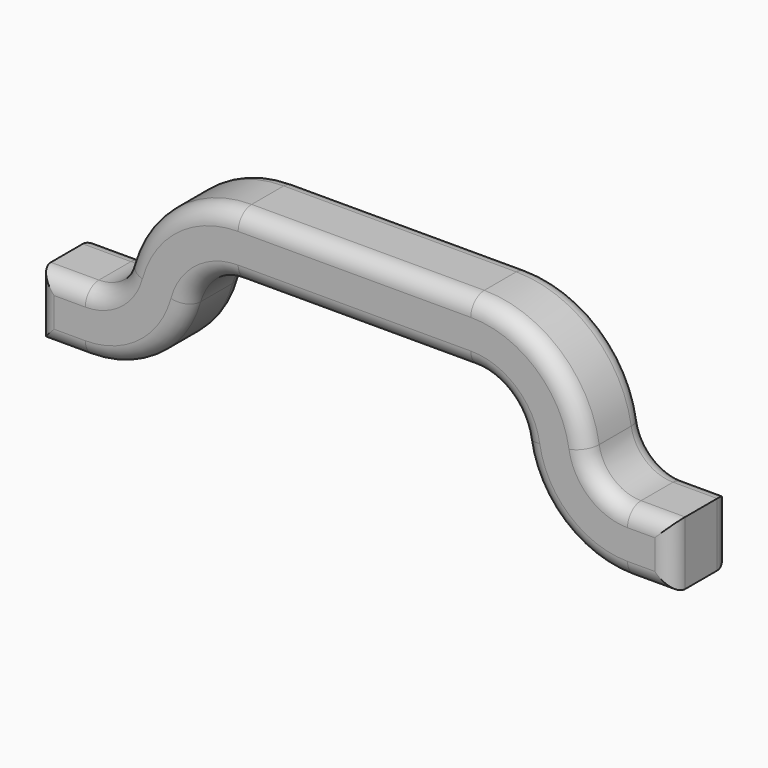
from build123d import *

# Parameters (mm, degrees)
F1_DEPTH = 22.1615
F2_R     = 5.08


# Not quite as in the source:
# - a feature names something its author has since deleted; it is built from what else it names


with BuildPart() as f1:
    # F0 (on Front) → F1 (new body)
    with BuildSketch(Plane.XZ):
        with BuildLine():
            Line((28.6224108991, 72.15352447), (-41.2275891009, 72.15352447))
            ThreePointArc((-41.2275891009, 72.15352447), (-62.3757268242, 65.0226226894), (-74.8879136272, 46.5418578033))
            ThreePointArc((-74.8879136272, 46.5418578033), (-79.4377997374, 39.8215796629), (-87.1280316368, 37.22852447))
            Line((-87.1280316368, 37.22852447), (-101.5525891009, 37.22852447))
            Line((-101.5525891009, 37.22852447), (-101.5525891009, 18.17852447))
            Line((-101.5525891009, 18.17852447), (-87.1280316368, 18.17852447))
            ThreePointArc((-87.1280316368, 18.17852447), (-67.9024518883, 24.6611624523), (-56.5277366129, 41.4618578033))
            ThreePointArc((-56.5277366129, 41.4618578033), (-50.8403789751, 49.8622054788), (-41.2275891009, 53.10352447))
            Line((-41.2275891009, 53.10352447), (28.6224108991, 53.10352447))
            ThreePointArc((28.6224108991, 53.10352447), (38.9482036141, 49.2864525593), (44.3084160673, 39.6708321623))
            ThreePointArc((44.3084160673, 39.6708321623), (55.0288409738, 20.4395913682), (75.6804264037, 12.8054475469))
            Line((75.6804264037, 12.8054475469), (88.9474108991, 12.8054475469))
            Line((88.9474108991, 12.8054475469), (88.9474108991, 31.8554475469))
            Line((88.9474108991, 31.8554475469), (75.6804264037, 31.8554475469))
            ThreePointArc((75.6804264037, 31.8554475469), (67.4197922317, 34.9091050754), (63.1316222691, 42.601601393))
            ThreePointArc((63.1316222691, 42.601601393), (51.3391548721, 63.7559662665), (28.6224108991, 72.15352447))
        make_face()
    extrude(amount=F1_DEPTH)

    # F2
    f2_edges = [f1.edges().sort_by_distance(p)[0] for p in [
        (88.947411, -22.1615, 22.330448),
        (82.313919, -22.1615, 31.855448),
        (67.419792, -22.1615, 34.909105),
        (51.339155, -22.1615, 63.755966),
        (-6.302589, -22.1615, 72.153524),
        (-62.375727, -22.1615, 65.022623),
        (-79.4378, -22.1615, 39.82158),
        (-94.34031, -22.1615, 37.228524),
        (-101.552589, -22.1615, 27.703524),
        (-94.34031, -22.1615, 18.178524),
        (-67.902452, -22.1615, 24.661162),
        (-50.840379, -22.1615, 49.862205),
        (-6.302589, -22.1615, 53.103524),
        (38.948204, -22.1615, 49.286453),
        (55.028841, -22.1615, 20.439591),
        (82.313919, -22.1615, 12.805448),
        (88.947411, 0, 22.330448),
        (82.313919, 0, 31.855448),
        (67.419792, 0, 34.909105),
        (51.339155, 0, 63.755966),
        (-6.302589, 0, 72.153524),
        (-62.375727, 0, 65.022623),
        (-79.4378, 0, 39.82158),
        (-94.34031, 0, 37.228524),
        (-101.552589, 0, 27.703524),
        (-94.34031, 0, 18.178524),
        (-67.902452, 0, 24.661162),
        (-50.840379, 0, 49.862205),
        (-6.302589, 0, 53.103524),
        (38.948204, 0, 49.286453),
        (55.028841, 0, 20.439591),
        (82.313919, 0, 12.805448),
    ]]
    fillet(f2_edges, radius=F2_R)


solid = f1.part
